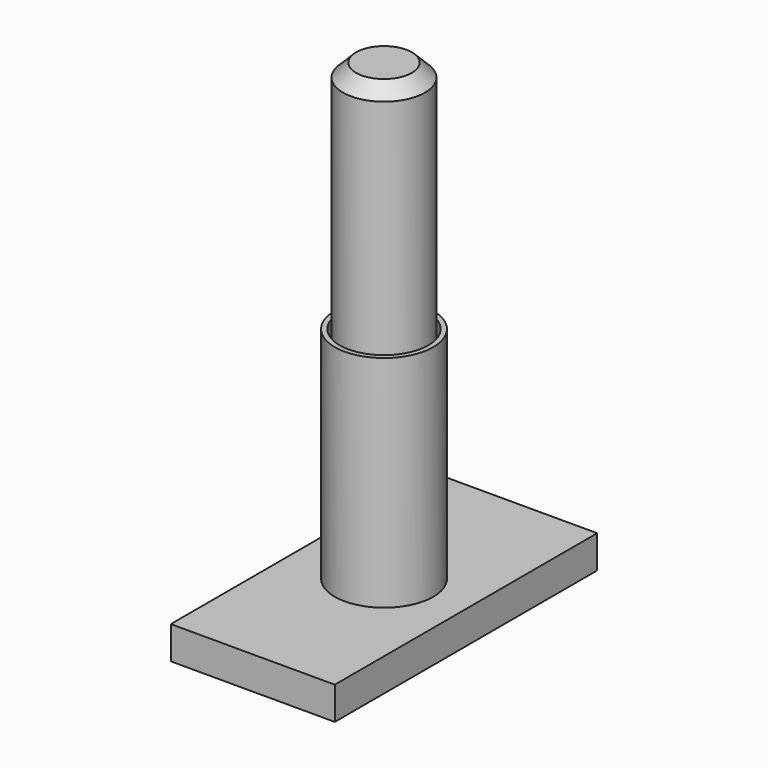
from build123d import *

# Parameters (mm, degrees)
F0_W         = 50
F0_H         = 100
F1_DEPTH     = 10
F2_R         = 15
F3_DEPTH     = 67
F4_T         = -1.5
F5_R         = 12.5
F6_DEPTH     = 147
F7_SIZE      = 4
F9_DEPTH     = 10
F10_W        = 5
F10_H        = 6
F11_DEPTH    = 20
F12_R        = 4
F13_R        = 4
F14_T1_DEPTH = 22.3205080757


# Not quite as in the source:
# - a fillet or chamfer that OpenCascade refuses, or shapes differently, is made with other operations: its cross-section is extruded or revolved along the edge and cut away or added


with BuildPart() as f1:
    # F0 (on Top) → F1 (new body)
    with BuildSketch(Plane.XY):
        Rectangle(F0_W, F0_H)
    extrude(amount=F1_DEPTH)

    # F2 (on face) → F3 (join)
    with BuildSketch(Plane.XY.offset(10)):
        Circle(F2_R)
    extrude(amount=F3_DEPTH)

    # F4
    f4_openings = [f1.faces().sort_by_distance(p)[0] for p in [
        (0, 0, 77),
    ]]
    offset(amount=F4_T, openings=f4_openings, kind=Kind.INTERSECTION)

    # F5 (on face) → F6 (join)
    with BuildSketch(Plane.XY.offset(1.5)):
        Circle(F5_R)
    extrude(amount=F6_DEPTH)

    # F7
    f7_edges = [f1.edges().sort_by_distance(p)[0] for p in [
        (-12.5, 0, 148.5),
    ]]
    chamfer(f7_edges, length=F7_SIZE)

    # F8 (on face) → F9 (join)
    with BuildSketch(Plane(origin=(0, 0, 0), x_dir=(1, 0, 0), z_dir=(0, 0, -1))):
        Polygon((2.5, 16), (0, 16), (-2.5, 16), (-2.5, 6), (2.5, 6), align=None)
    extrude(amount=F9_DEPTH)

    # F10 (on face) → F11 (join)
    with BuildSketch(Plane(origin=(0, -6, 0), x_dir=(-1, 0, 0), z_dir=(0, 1, 0))):
        with Locations((0, -7)):
            Rectangle(F10_W, F10_H)
    extrude(amount=F11_DEPTH)

    # F12
    f12_edges = [f1.edges().sort_by_distance(p)[0] for p in [
        (0, 14, -10),
    ]]
    fillet(f12_edges, radius=F12_R)

    # F13
    f13_edges = [f1.edges().sort_by_distance(p)[0] for p in [
        (0, -16, -10),
    ]]
    fillet(f13_edges, radius=F13_R)

    # F14: fillet of radius 4 on 1 edges, made by hand

    # F14_s2 → F14_t1 (cut)
    with BuildSketch(Plane.YZ.offset(-11.1602540378)):
        with BuildLine():
            ThreePointArc((14, -6), (12.5358983849, -4.5358983849), (10.5358983849, -4))
            Line((10.5358983849, -4), (14, -4))
            Line((14, -4), (14, -6))
        make_face()
    extrude(amount=F14_T1_DEPTH, mode=Mode.SUBTRACT)


solid = f1.part
